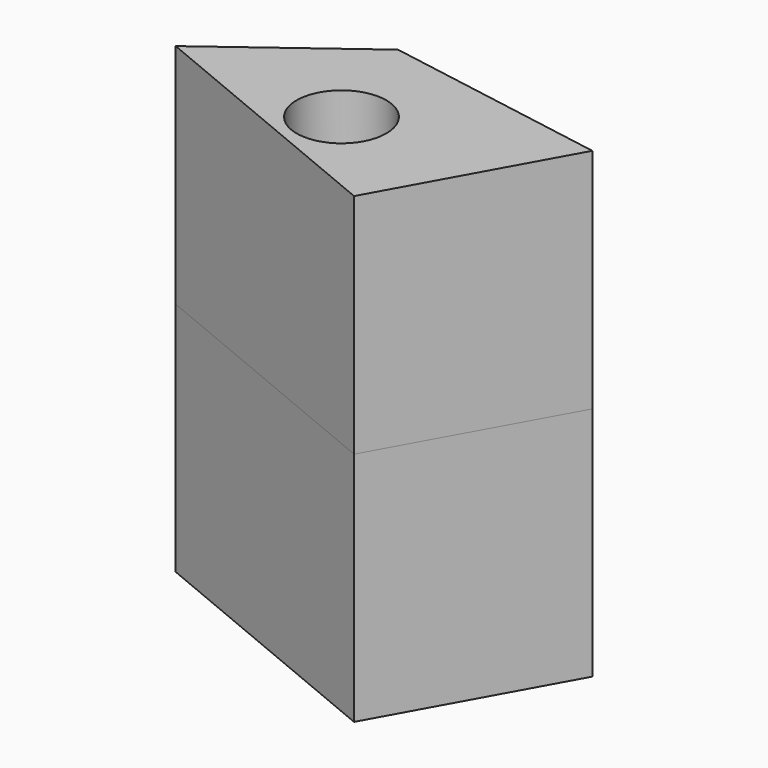
from build123d import *

# Parameters (mm, degrees)
F1_DEPTH = 83
F3_DEPTH = 80
F4_R     = 15.7967970704
F5_DEPTH = 261


# Not quite as in the source:
# - the program builds the solid bodies; features that only make, move or delete a surface that nothing else refers to are left out


with BuildPart() as f1:
    # F0 (on Top) → F1 (new body)
    with BuildSketch(Plane.XY):
        Polygon((-20.6632390618, 40.9574918449), (-69.738432765, 4.4278339483), (24.3531055748, -34.6847251058), (58.6688406765, 27.3049920797), align=None)
    extrude(amount=F1_DEPTH)


with BuildPart() as f3:
    # F3 (new): a face of the model
    f3_faces = [f1.part.faces().sort_by_distance(p)[0] for p in [
        (-0.5558487056, 7.3902608485, 83),
    ]]
    extrude(f3_faces, amount=F3_DEPTH)

    # F4 (on face) → F5 (cut)
    with BuildSketch(Plane.XY.offset(163)):
        with Locations((-7.8215794638, 0)):
            Circle(F4_R)
    extrude(amount=-F5_DEPTH, mode=Mode.SUBTRACT)


solid = Compound([f1.part, f3.part])
